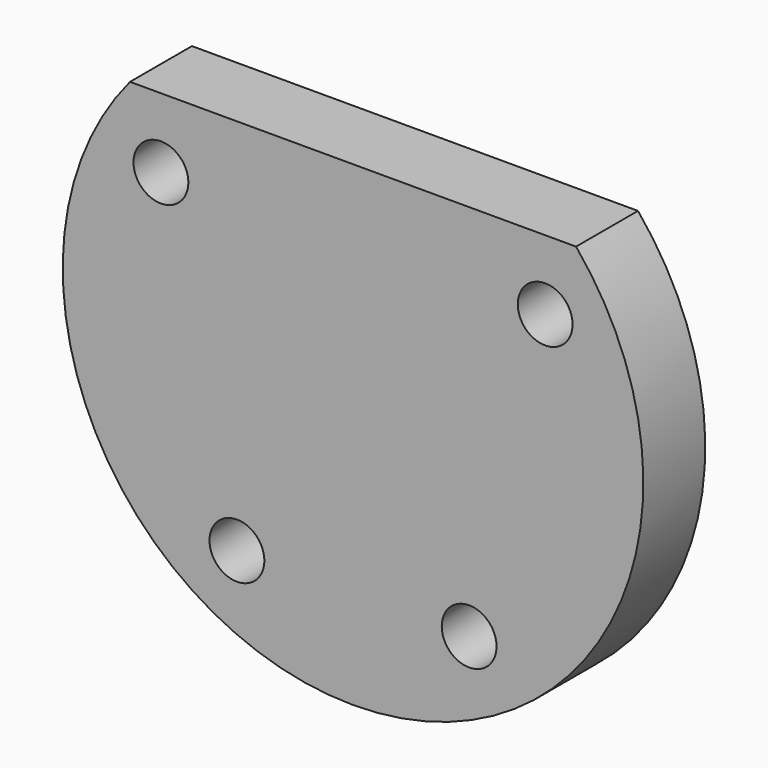
from build123d import *

# Parameters (mm, degrees)
F1_DEPTH = 6.35
F3_D     = 4.4958


with BuildPart() as f1:
    # F0 (on Front) → F1 (new body)
    with BuildSketch(Plane.XZ):
        with BuildLine():
            Line((18.2969275085, 15.24), (-18.2969275085, 15.24))
            ThreePointArc((-18.2969275085, 15.24), (0, -23.8125), (18.2969275085, 15.24))
        make_face()
    extrude(amount=F1_DEPTH)

    # F3 (through all)
    with Locations(Plane.XZ.offset(6.35)):
        with Locations((-15.7602855304, 9.525), (15.7602855304, 9.525), (-9.525, -15.7602855304), (9.525, -15.7602855304)):
            Hole(F3_D / 2)


solid = f1.part
